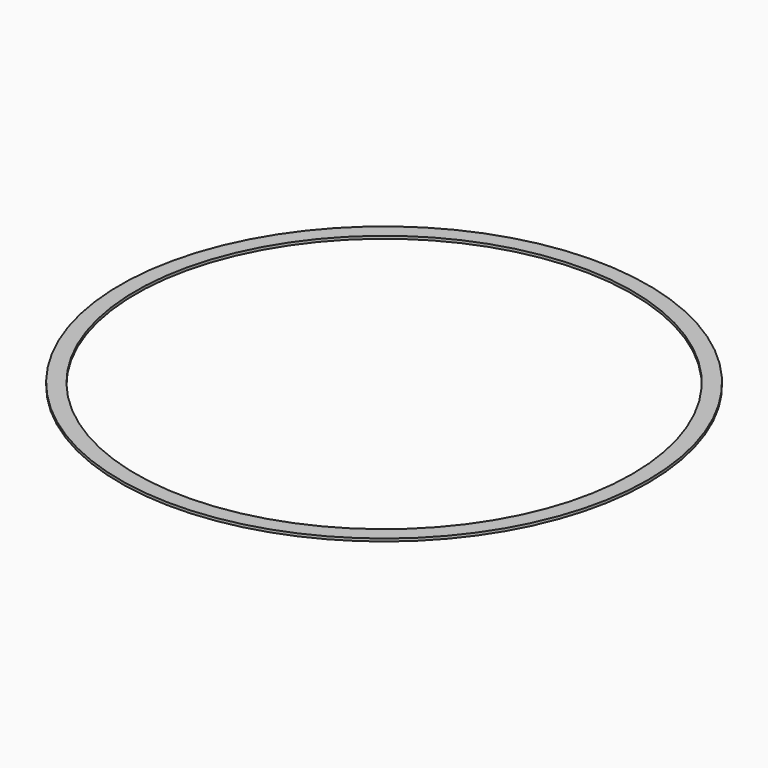
from build123d import *

# Parameters (mm, degrees)
F0_R     = 422.34231
F0_R_2   = 396.94231
F1_DEPTH = 4.2333333333


# Not quite as in the source:
# - a length typed as a fraction of an inch, garbled in the dataset ("3 / 203.2 mm" for 3/8 in), is restored


with BuildPart() as f1:
    # F0 (on Top) → F1 (new body)
    with BuildSketch(Plane.XY):
        Circle(F0_R)
        Circle(F0_R_2, mode=Mode.SUBTRACT)
    extrude(amount=F1_DEPTH)


solid = f1.part
